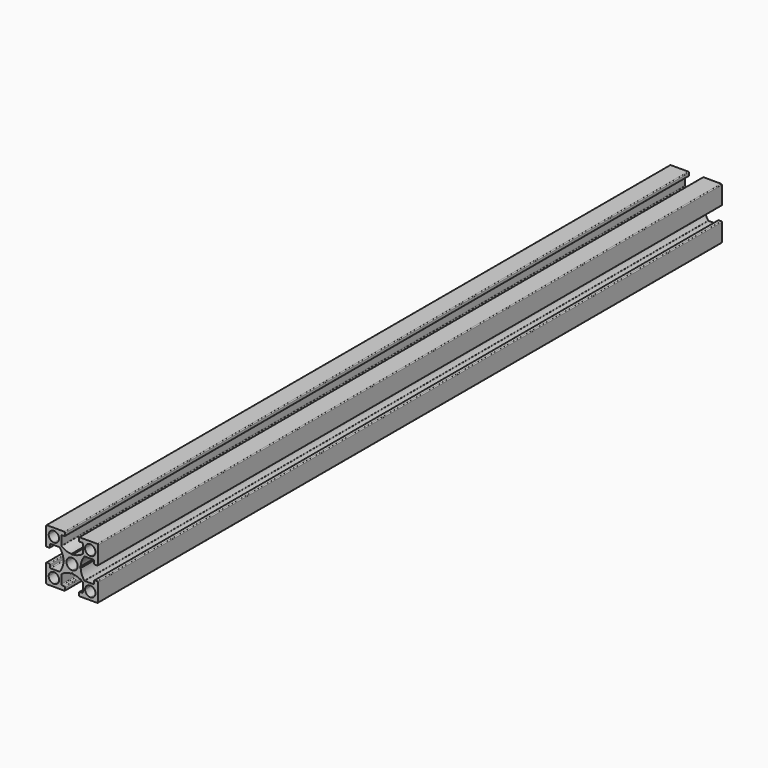
from build123d import *

# Parameters (mm, degrees)
F1_DEPTH = 300


# Not quite as in the source:
# - ends of sketch curves that miss each other by under 0.0002 mm in the source are joined


with BuildPart() as f1:
    # F0 (on Front) → F1 (new body)
    with BuildSketch(Plane.XZ):
        with BuildLine():
            ThreePointArc((0, 2.15), (1.5202795796, 1.5202795796), (2.15, 0))
            Line((2.15, 0), (3, 0))
            Line((3, 0), (3.307278, 0.307278))
            ThreePointArc((3.307278, 0.307278), (3.7143803747, 2.2820219924), (4.7078187099, 4.0365664363))
            ThreePointArc((4.7078187099, 4.0365664363), (4.812308461, 4.1201573706), (4.94275, 4.15))
            Line((4.94275, 4.15), (8.2, 4.15))
            ThreePointArc((8.2, 4.15), (8.4121320344, 4.0621320344), (8.5, 3.85))
            Line((8.5, 3.85), (8.5, 2.95))
            ThreePointArc((8.5, 2.95), (8.5878679656, 2.7378679656), (8.8, 2.65))
            Line((8.8, 2.65), (9.7, 2.65))
            ThreePointArc((9.7, 2.65), (9.9121320344, 2.7378679656), (10, 2.95))
            Line((10, 2.95), (10, 9.7))
            ThreePointArc((10, 9.7), (9.9121320344, 9.9121320344), (9.7, 10))
            Line((9.7, 10), (2.95, 10))
            ThreePointArc((2.95, 10), (2.7378679656, 9.9121320344), (2.65, 9.7))
            Line((2.65, 9.7), (2.65, 8.8))
            ThreePointArc((2.65, 8.8), (2.7378679656, 8.5878679656), (2.95, 8.5))
            Line((2.95, 8.5), (3.85, 8.5))
            ThreePointArc((3.85, 8.5), (4.0621320344, 8.4121320344), (4.15, 8.2))
            Line((4.15, 8.2), (4.15, 4.94275))
            ThreePointArc((4.15, 4.94275), (4.1201572004, 4.8123081084), (4.036566086, 4.7078178916))
            ThreePointArc((4.036566086, 4.7078178916), (2.2820216259, 3.7143802371), (0.3072779813, 3.3072783955))
            Line((0.3072779813, 3.3072783955), (0, 3))
            Line((0, 3), (0, 2.15))
        make_face()
        with BuildLine():
            ThreePointArc((7, 9), (8.4142135624, 8.4142135624), (9, 7))
            ThreePointArc((9, 7), (8.4142135624, 5.5857864376), (7, 5))
            ThreePointArc((7, 5), (5.5857864376, 5.5857864376), (5, 7))
            ThreePointArc((5, 7), (5.5857864376, 8.4142135624), (7, 9))
        make_face(mode=Mode.SUBTRACT)
        with BuildLine():
            Line((3, 0), (2.15, 0))
            ThreePointArc((2.15, 0), (1.5202795796, -1.5202795796), (0, -2.15))
            Line((0, -2.15), (0, -3))
            Line((0, -3), (0.307278, -3.307277))
            ThreePointArc((0.307278, -3.307277), (2.2820216259, -3.7143792371), (4.036565823, -4.7078172229))
            ThreePointArc((4.036565823, -4.7078172229), (4.1201572004, -4.8123071084), (4.15, -4.942749))
            Line((4.15, -4.942749), (4.15, -8.2))
            ThreePointArc((4.15, -8.2), (4.0621320344, -8.4121320344), (3.85, -8.5))
            Line((3.85, -8.5), (2.95, -8.5))
            ThreePointArc((2.95, -8.5), (2.7378679656, -8.5878679656), (2.65, -8.8))
            Line((2.65, -8.8), (2.65, -9.7))
            ThreePointArc((2.65, -9.7), (2.7378679656, -9.9121320344), (2.95, -10))
            Line((2.95, -10), (9.7, -10))
            ThreePointArc((9.7, -10), (9.9121320344, -9.9121320344), (10, -9.7))
            Line((10, -9.7), (10, -2.95))
            ThreePointArc((10, -2.95), (9.9121320344, -2.7378679656), (9.7, -2.65))
            Line((9.7, -2.65), (8.8, -2.65))
            ThreePointArc((8.8, -2.65), (8.5878679656, -2.7378679656), (8.5, -2.95))
            Line((8.5, -2.95), (8.5, -3.85))
            ThreePointArc((8.5, -3.85), (8.4121320344, -4.0621320344), (8.2, -4.15))
            Line((8.2, -4.15), (4.94275, -4.15))
            ThreePointArc((4.94275, -4.15), (4.8123081084, -4.1201572004), (4.7078178916, -4.036566086))
            ThreePointArc((4.7078178916, -4.036566086), (3.7143800615, -2.2820211583), (3.3072783483, -0.3072769835))
            Line((3.3072783483, -0.3072769835), (3, 0))
        make_face()
        with BuildLine():
            ThreePointArc((7, -5), (8.4142135624, -5.5857864376), (9, -7))
            ThreePointArc((9, -7), (8.4142135624, -8.4142135624), (7, -9))
            ThreePointArc((7, -9), (5.5857864376, -8.4142135624), (5, -7))
            ThreePointArc((5, -7), (5.5857864376, -5.5857864376), (7, -5))
        make_face(mode=Mode.SUBTRACT)
        with BuildLine():
            Line((0, -3), (0, -2.15))
            ThreePointArc((0, -2.15), (-1.5202795796, -1.5202795796), (-2.15, 0))
            Line((-2.15, 0), (-3, 0))
            Line((-3, 0), (-3.307277, -0.307277))
            ThreePointArc((-3.307277, -0.307277), (-3.7143790615, -2.2820211583), (-4.7078172229, -4.036565823))
            ThreePointArc((-4.7078172229, -4.036565823), (-4.8123071084, -4.1201572004), (-4.942749, -4.15))
            Line((-4.942749, -4.15), (-8.2, -4.15))
            ThreePointArc((-8.2, -4.15), (-8.4121320344, -4.0621320344), (-8.5, -3.85))
            Line((-8.5, -3.85), (-8.5, -2.95))
            ThreePointArc((-8.5, -2.95), (-8.5878679656, -2.7378679656), (-8.8, -2.65))
            Line((-8.8, -2.65), (-9.7, -2.65))
            ThreePointArc((-9.7, -2.65), (-9.9121320344, -2.7378679656), (-10, -2.95))
            Line((-10, -2.95), (-10, -9.7))
            ThreePointArc((-10, -9.7), (-9.9121320344, -9.9121320344), (-9.7, -10))
            Line((-9.7, -10), (-2.95, -10))
            ThreePointArc((-2.95, -10), (-2.7378679656, -9.9121320344), (-2.65, -9.7))
            Line((-2.65, -9.7), (-2.65, -8.8))
            ThreePointArc((-2.65, -8.8), (-2.7378679656, -8.5878679656), (-2.95, -8.5))
            Line((-2.95, -8.5), (-3.85, -8.5))
            ThreePointArc((-3.85, -8.5), (-4.0621320344, -8.4121320344), (-4.15, -8.2))
            Line((-4.15, -8.2), (-4.15, -4.942749))
            ThreePointArc((-4.15, -4.942749), (-4.1201572004, -4.8123071084), (-4.036566086, -4.7078168916))
            ThreePointArc((-4.036566086, -4.7078168916), (-2.2820211583, -3.7143790615), (-0.3072769835, -3.3072773483))
            Line((-0.3072769835, -3.3072773483), (0, -3))
        make_face()
        with BuildLine():
            ThreePointArc((-7, -9), (-8.4142135624, -8.4142135624), (-9, -7))
            ThreePointArc((-9, -7), (-8.4142135624, -5.5857864376), (-7, -5))
            ThreePointArc((-7, -5), (-5.5857864376, -5.5857864376), (-5, -7))
            ThreePointArc((-5, -7), (-5.5857864376, -8.4142135624), (-7, -9))
        make_face(mode=Mode.SUBTRACT)
        with BuildLine():
            ThreePointArc((-2.15, 0), (-1.5202795796, 1.5202795796), (0, 2.15))
            Line((0, 2.15), (0, 3))
            Line((0, 3), (-0.307277, 3.307278))
            ThreePointArc((-0.307277, 3.307278), (-2.2820211583, 3.7143800615), (-4.036565823, 4.7078182229))
            ThreePointArc((-4.036565823, 4.7078182229), (-4.1201572004, 4.8123081084), (-4.15, 4.94275))
            Line((-4.15, 4.94275), (-4.15, 8.2))
            ThreePointArc((-4.15, 8.2), (-4.0621320344, 8.4121320344), (-3.85, 8.5))
            Line((-3.85, 8.5), (-2.95, 8.5))
            ThreePointArc((-2.95, 8.5), (-2.7378679656, 8.5878679656), (-2.65, 8.8))
            Line((-2.65, 8.8), (-2.65, 9.7))
            ThreePointArc((-2.65, 9.7), (-2.7378679656, 9.9121320344), (-2.95, 10))
            Line((-2.95, 10), (-9.7, 10))
            ThreePointArc((-9.7, 10), (-9.9121320344, 9.9121320344), (-10, 9.7))
            Line((-10, 9.7), (-10, 2.95))
            ThreePointArc((-10, 2.95), (-9.9121320344, 2.7378679656), (-9.7, 2.65))
            Line((-9.7, 2.65), (-8.8, 2.65))
            ThreePointArc((-8.8, 2.65), (-8.5878679656, 2.7378679656), (-8.5, 2.95))
            Line((-8.5, 2.95), (-8.5, 3.85))
            ThreePointArc((-8.5, 3.85), (-8.4121320344, 4.0621320344), (-8.2, 4.15))
            Line((-8.2, 4.15), (-4.942749, 4.15))
            ThreePointArc((-4.942749, 4.15), (-4.812307461, 4.1201573706), (-4.7078173786, 4.0365666993))
            ThreePointArc((-4.7078173786, 4.0365666993), (-3.7143793747, 2.2820219924), (-3.3072773955, 0.3072779813))
            Line((-3.3072773955, 0.3072779813), (-3, 0))
            Line((-3, 0), (-2.15, 0))
        make_face()
        with BuildLine():
            ThreePointArc((-7, 5), (-8.4142135624, 5.5857864376), (-9, 7))
            ThreePointArc((-9, 7), (-8.4142135624, 8.4142135624), (-7, 9))
            ThreePointArc((-7, 9), (-5.5857864376, 8.4142135624), (-5, 7))
            ThreePointArc((-5, 7), (-5.5857864376, 5.5857864376), (-7, 5))
        make_face(mode=Mode.SUBTRACT)
    extrude(amount=F1_DEPTH)


solid = f1.part
